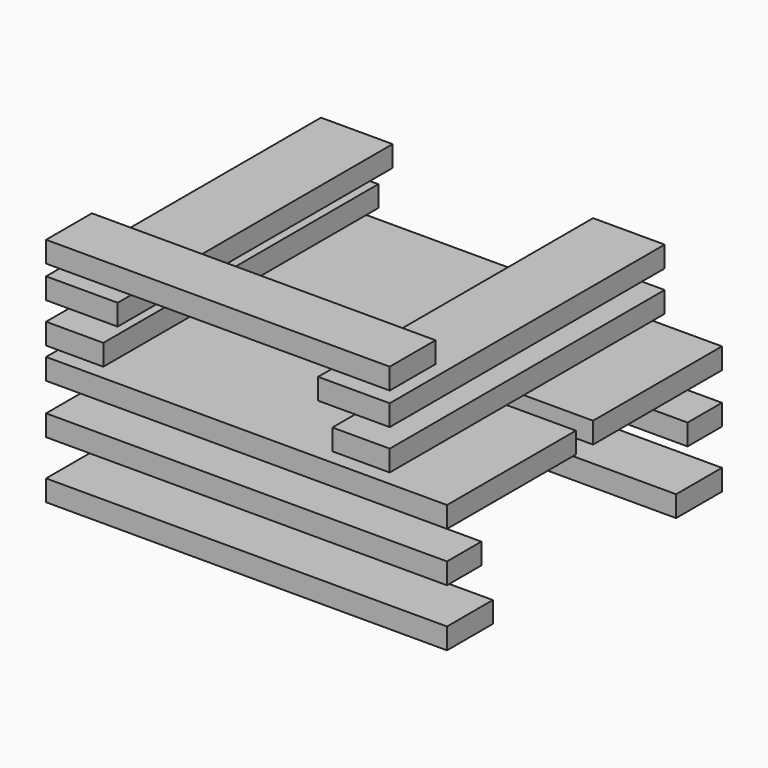
from build123d import *

# Parameters (mm, degrees)
F0_W          = 63.5
F0_H          = 18.6436
F1_DEPTH      = 304.8
F0_W_2        = 50.8
F0_W_3        = 355.6
F3_DEPTH      = 81.5790404614
F4_W          = 50.8
F4_H          = 18.6436
F5_DEPTH      = 177.8
F4_W_2        = 38.1
F6_W          = 50.8
F6_H          = 18.6436
F7_DEPTH      = 127
F7_DEPTH_BACK = 177.8


with BuildPart() as f1:
    # F0 (on Front) → F1 (new body)
    with BuildSketch(Plane.XZ):
        with Locations((-146.05, 62.9344404614)):
            Rectangle(F0_W, F0_H)
    extrude(amount=F1_DEPTH)


with BuildPart() as f1b:
    # F0 (on Front) → F1, piece 2 (new body)
    with BuildSketch(Plane.XZ):
        with Locations((-152.4, 27.5055062211)):
            Rectangle(F0_W_2, F0_H)
    extrude(amount=F1_DEPTH)


with BuildPart() as f1c:
    # F0 (on Front) → F1, piece 3 (new body)
    with BuildSketch(Plane.XZ):
        Rectangle(F0_W_3, F0_H)
    extrude(amount=F1_DEPTH)

    # F2 (on face) → F3 (cut, through all)
    with BuildSketch(Plane(origin=(0, 0, -9.3218), x_dir=(1, 0, 0), z_dir=(0, 0, -1))):
        with BuildLine():
            Line((177.8, 161.925), (-142.875, 161.925))
            ThreePointArc((-142.875, 161.925), (-152.4, 152.4), (-142.875, 142.875))
            Line((-142.875, 142.875), (177.8, 142.875))
            Line((177.8, 142.875), (177.8, 161.925))
        make_face()
    extrude(amount=-F3_DEPTH, mode=Mode.SUBTRACT)


with BuildPart() as f1d:
    # F0 (on Front) → F1, piece 4 (new body)
    with BuildSketch(Plane.XZ):
        with Locations((101.6, 27.5055062211)):
            Rectangle(F0_W_2, F0_H)
    extrude(amount=F1_DEPTH)


with BuildPart() as f1e:
    # F0 (on Front) → F1, piece 5 (new body)
    with BuildSketch(Plane.XZ):
        with Locations((95.25, 62.9344404614)):
            Rectangle(F0_W, F0_H)
    extrude(amount=F1_DEPTH)


with BuildPart() as f5:
    # F4 (on Right) → F5 (new body, symmetric)
    with BuildSketch(Plane.YZ):
        with Locations((-25.4, -94.8436)):
            Rectangle(F4_W, F4_H)
    extrude(amount=F5_DEPTH, both=True)


with BuildPart() as f5b:
    # F4 (on Right) → F5, piece 2 (new body, symmetric)
    with BuildSketch(Plane.YZ):
        with Locations((-279.4, -94.8436)):
            Rectangle(F4_W, F4_H)
    extrude(amount=F5_DEPTH, both=True)


with BuildPart() as f5c:
    # F4 (on Right) → F5, piece 3 (new body, symmetric)
    with BuildSketch(Plane.YZ):
        with Locations((-285.75, -44.0436)):
            Rectangle(F4_W_2, F4_H)
    extrude(amount=F5_DEPTH, both=True)


with BuildPart() as f5d:
    # F4 (on Right) → F5, piece 4 (new body, symmetric)
    with BuildSketch(Plane.YZ):
        with Locations((-19.05, -44.0436)):
            Rectangle(F4_W_2, F4_H)
    extrude(amount=F5_DEPTH, both=True)


with BuildPart() as f7:
    # F6 (on Right) → F7 (new body, two sides)
    with BuildSketch(Plane.YZ) as f7_sk:
        with Locations((-279.4, 91.4935171604)):
            Rectangle(F6_W, F6_H)
    extrude(amount=F7_DEPTH)
    extrude(f7_sk.sketch, amount=-F7_DEPTH_BACK)


solid = Compound([f1.part, f1b.part, f1c.part, f1d.part, f1e.part, f5.part, f5b.part, f5c.part, f5d.part, f7.part])
